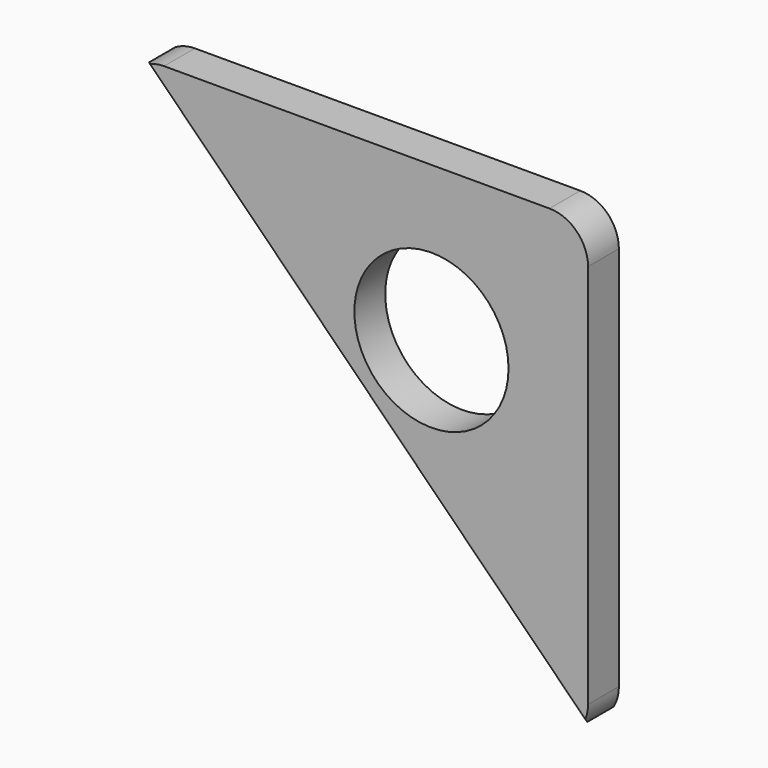
from build123d import *

# Parameters (mm, degrees)
F0_R        = 50
F1_DEPTH    = 25
F2_SIZE     = 10
F3_T1_DEPTH = 47.2159409701


# Not quite as in the source:
# - a fillet or chamfer that OpenCascade refuses, or shapes differently, is made with other operations: its cross-section is extruded or revolved along the edge and cut away or added


with BuildPart() as f1:
    # F0 (on Front) → F1 (new body)
    with BuildSketch(Plane.XZ):
        with BuildLine():
            Line((51.0779787002, 143.0251310061), (-198.9220212998, 143.0251310061))
            ThreePointArc((-198.9220212998, 143.0251310061), (-208.4891071089, 141.1221193189), (-216.5996908295, 135.7028005358))
            Line((-216.5996908295, 135.7028005358), (68.7556482299, -149.6525385235))
            ThreePointArc((68.7556482299, -149.6525385235), (74.174967013, -141.541954803), (76.0779787002, -131.9748689939))
            Line((76.0779787002, -131.9748689939), (76.0779787002, 118.0251310061))
            ThreePointArc((76.0779787002, 118.0251310061), (68.7556482299, 135.7028005358), (51.0779787002, 143.0251310061))
        make_face()
        with Locations((-25.4944633545, 42.9471413087)):
            Circle(F0_R, mode=Mode.SUBTRACT)
    extrude(amount=F1_DEPTH)

    # F2
    f2_edges = [f1.edges().sort_by_distance(p)[0] for p in [
        (-73.922021, -25, -6.974869),
    ]]
    chamfer(f2_edges, length=F2_SIZE)

    # F3: chamfer of 5 on 2 edges, made by hand

    # F3_s2 → F3_t1 (cut)
    with BuildSketch(Plane.XZ.offset(-16.1079704851)):
        with BuildLine():
            Line((64.7710426378, -145.6679329315), (72.6137260047, -144.6717815335))
            ThreePointArc((72.6137260047, -144.6717815335), (70.8856590953, -147.2279276171), (68.7556482299, -149.6525385235))
            Line((68.7556482299, -149.6525385235), (64.7710426378, -145.6679329315))
        make_face()
        with BuildLine():
            Line((-211.6189338394, 139.5608783106), (-212.6150852374, 131.7181949438))
            Line((-212.6150852374, 131.7181949438), (-216.5996908295, 135.7028005358))
            ThreePointArc((-216.5996908295, 135.7028005358), (-214.1750799231, 137.8328114012), (-211.6189338394, 139.5608783106))
        make_face()
    extrude(amount=F3_T1_DEPTH, mode=Mode.SUBTRACT)


solid = f1.part
